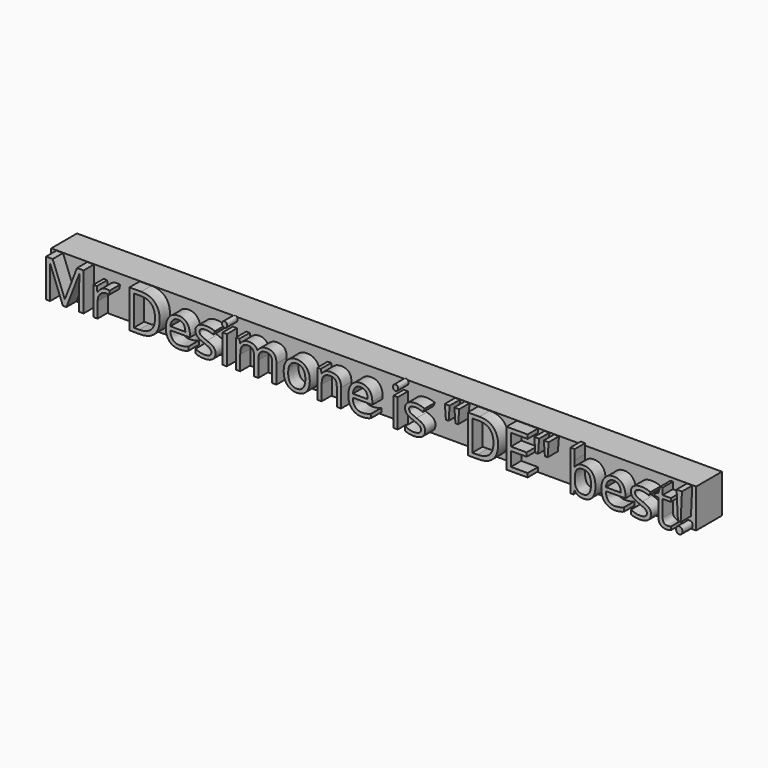
from build123d import *

# Parameters (mm, degrees)
F0_TEXT_SIZE = 10.4463608673
F1_DEPTH     = 2.54
F2_W         = 127
F2_H         = 7.62
F3_DEPTH     = 6.35


# Not quite as in the source:
# - Text() gives the source's letters only with a copy of the font that has no kerning and outlines rounded to 1/6400 em; it was checked with that copy


with BuildPart() as f1:
    # F0 (on Front) → F1 (new body)
    with BuildSketch(Plane.XZ):
        with Locations((0, -7.5213798244)):
            Text('Mr Desimone is "DE" best!', F0_TEXT_SIZE, font='Open Sans', text_align=(TextAlign.LEFT, TextAlign.BOTTOM))
    extrude(amount=F1_DEPTH)


with BuildPart() as f3:
    # F2 (on Front) → F3 (new body)
    with BuildSketch(Plane.XZ):
        with Locations((63.5, -3.81)):
            Rectangle(F2_W, F2_H)
    extrude(amount=-F3_DEPTH)


solid = Compound([f1.part, f3.part])
